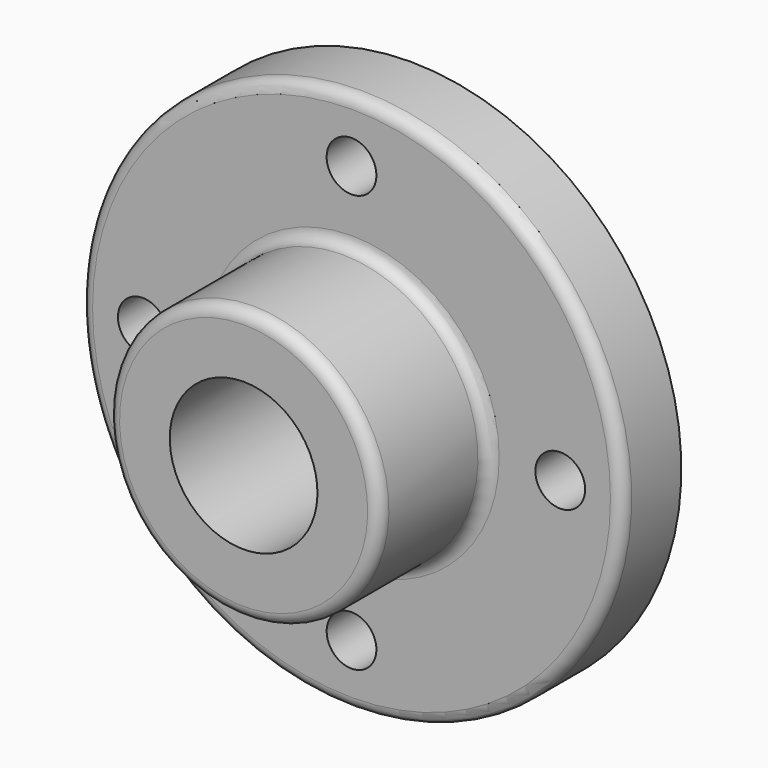
from build123d import *

# Parameters (mm, degrees)
F2_R            = 6.4164417579
F3_DEPTH        = 19.051
F3_COPIES_COUNT = 4
F4_R            = 3.048


# Not quite as in the source:
# - a pattern or mirror of a feature is missing from the dataset's text; its kind, count and spacing are read off the source's solid


with BuildPart() as f1:
    # F0 (on Right) → F1 (revolve)
    with BuildSketch(Plane.YZ):
        Polygon((-53.848, 19.05), (0, 19.05), (0, 69.85), (-19.05, 69.85), (-19.05, 35.052), (-53.848, 35.052), align=None)
    revolve(axis=Axis((0, -58.1718310714, 0), (0, -1, 0)))

    # F2 (on face) → F3 (cut, through all)
    with BuildSketch(Plane.XZ.offset(19.05)):
        with Locations((-53.848, 0)):
            Circle(F2_R)
    f3 = extrude(amount=-F3_DEPTH, mode=Mode.SUBTRACT)

    # F3_copies: F3 ×4 about axis
    f3_copies_axis = Axis((0, 0, 0), (0, 1, 0))
    for i in range(1, F3_COPIES_COUNT):
        add(f3.rotate(f3_copies_axis, i * 360 / F3_COPIES_COUNT), mode=Mode.SUBTRACT)

    # F4
    f4_edges = [f1.edges().sort_by_distance(p)[0] for p in [
        (0, -53.848, -35.052),
        (0, -19.05, -35.052),
        (0, -19.05, -69.85),
    ]]
    fillet(f4_edges, radius=F4_R)


solid = f1.part
